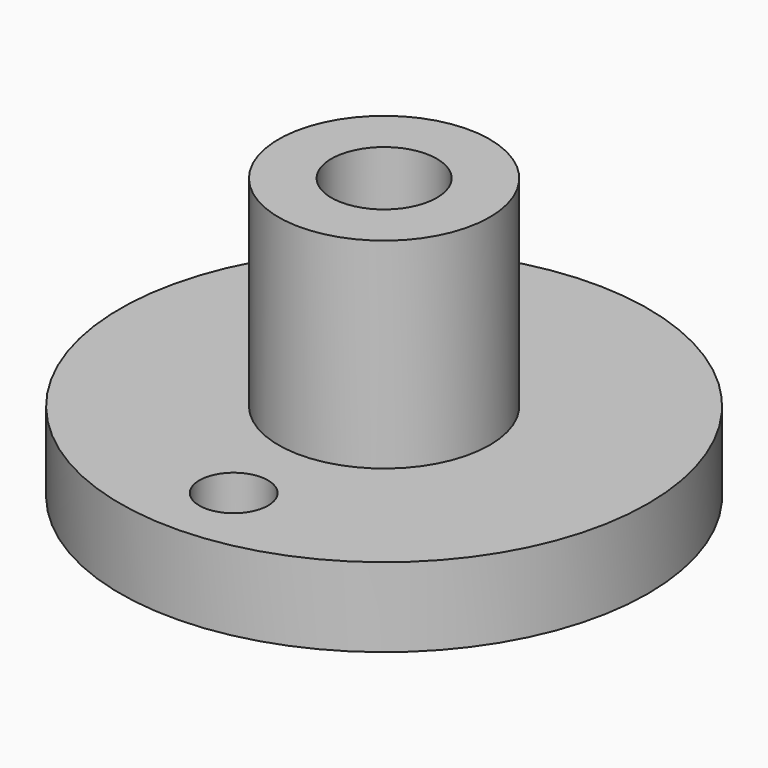
from build123d import *

# Parameters (mm, degrees)
F0_R     = 5
F0_R_2   = 1
F1_DEPTH = 1.5
F2_R     = 2
F2_R_2   = 1
F3_DEPTH = 3.8
F4_R     = 0.6498381819
F5_DEPTH = 1.5


# Not quite as in the source:
# - a feature names something its author has since deleted; it is built from what else it names


with BuildPart() as f1:
    # F0 (on Top) → F1 (new body)
    with BuildSketch(Plane.XY):
        Circle(F0_R)
        Circle(F0_R_2, mode=Mode.SUBTRACT)
    extrude(amount=F1_DEPTH)

    # F2 (on face) → F3 (join)
    with BuildSketch(Plane.XY.offset(1.5)):
        Circle(F2_R)
        Circle(F2_R_2, mode=Mode.SUBTRACT)
    extrude(amount=F3_DEPTH)

    # F4 (on Top) → F5 (cut, through all)
    with BuildSketch(Plane.XY):
        with Locations((0, -3.5616646055)):
            Circle(F4_R)
    extrude(amount=F5_DEPTH, mode=Mode.SUBTRACT)


solid = f1.part
